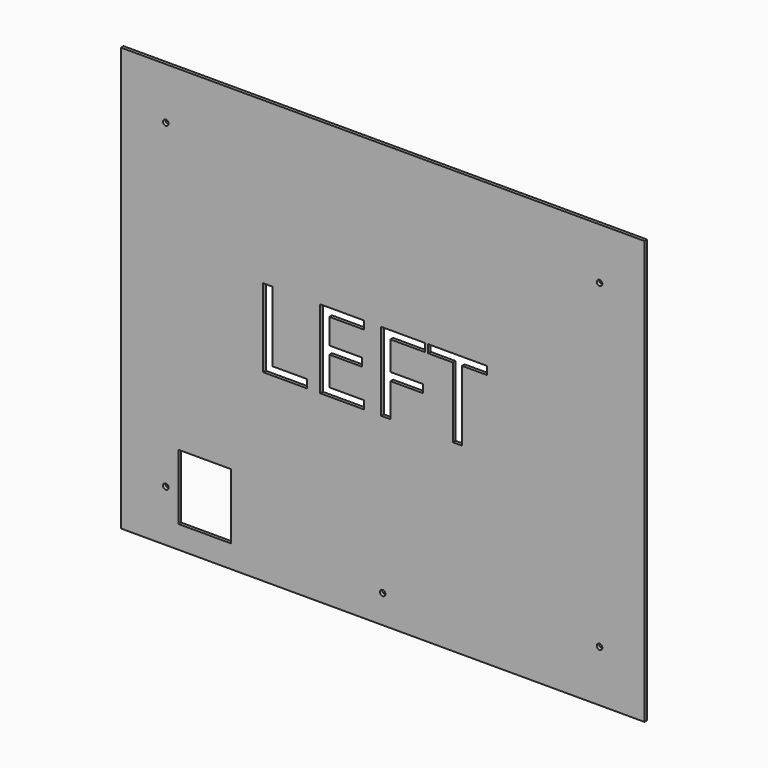
from build123d import *

# Parameters (mm, degrees)
F0_W         = 508.25
F0_H         = 411
F1_DEPTH     = 3.175
F2_TEXT_SIZE = 106.5619574446
F3_DEPTH     = 25
F4_R         = 2.7
F5_DEPTH     = 25
F7_W         = 50.8
F7_H         = 63.5
F8_DEPTH     = 25


# Not quite as in the source:
# - Text() gives the source's letters only with a copy of the font that has no kerning and outlines rounded to 1/6400 em; it was checked with that copy


with BuildPart() as f1:
    # F0 (on Front) → F1 (new body)
    with BuildSketch(Plane.XZ):
        Rectangle(F0_W, F0_H)
    extrude(amount=F1_DEPTH)

    # F2 (on face) → F3 (cut)
    with BuildSketch(Plane.XZ.offset(3.175)):
        with Locations((-126.433506608, -27.015702799)):
            Text('LEFT', F2_TEXT_SIZE, font='Open Sans', text_align=(TextAlign.LEFT, TextAlign.BOTTOM))
    extrude(amount=-F3_DEPTH, mode=Mode.SUBTRACT)

    # F4 (on face) → F5 (cut)
    with BuildSketch(Plane.XZ.offset(3.175)):
        with Locations((-210.525, 155.5)):
            Circle(F4_R)
        with Locations((-210.525, -155.5)):
            Circle(F4_R)
        with Locations((210.525, 155.5)):
            Circle(F4_R)
        with Locations((210.525, -155.5)):
            Circle(F4_R)
        with Locations((-0.025, -178)):
            Circle(F4_R)
    extrude(amount=-F5_DEPTH, mode=Mode.SUBTRACT)

    # F7 (on face) → F8 (cut)
    with BuildSketch(Plane.XZ.offset(3.175)):
        with Locations((-172.825, -151.75)):
            Rectangle(F7_W, F7_H)
    extrude(amount=-F8_DEPTH, mode=Mode.SUBTRACT)


solid = f1.part
